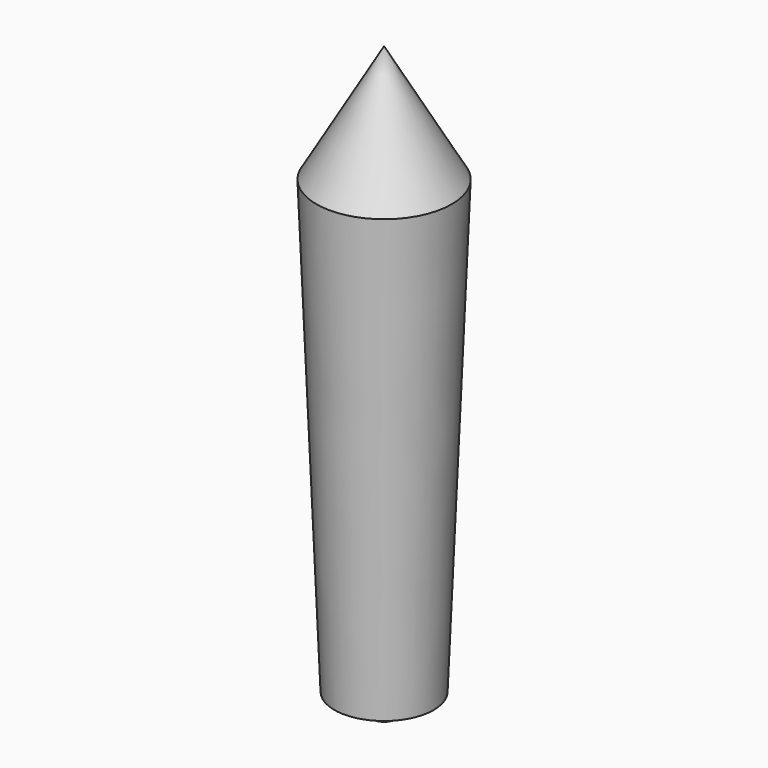
from build123d import *

# Parameters (mm, degrees)
F0_W = 4.4006289305
F0_H = 4
F2_R = 3.99999


# Not quite as in the source:
# - a fillet or chamfer is up to 0.001 mm smaller than in the source, because OpenCascade refuses the exact size


with BuildPart() as f1:
    # F0 (on Front) → F1 (revolve)
    with BuildSketch(Plane.XZ):
        Polygon((12, 29.6243050845), (0, 50.4089147754), (0, 29.6243050845), align=None)
        Polygon((8.801257861, -50.3756949155), (12, 29.6243050845), (0, 29.6243050845), (0, -50.3756949155), (4.4006289305, -50.3756949155), align=None)
        with Locations((2.2003144653, -52.3756949155)):
            Rectangle(F0_W, F0_H)
    revolve(axis=Axis((0, 0, -1.98339007), (0, 0, -1)))

    # F2 (radius 4 in the source; OpenCascade refuses exactly that, so slightly less here)
    f2_edges = [f1.edges().sort_by_distance(p)[0] for p in [
        (-4.400629, 0, -54.375695),
    ]]
    fillet(f2_edges, radius=F2_R)


solid = f1.part
